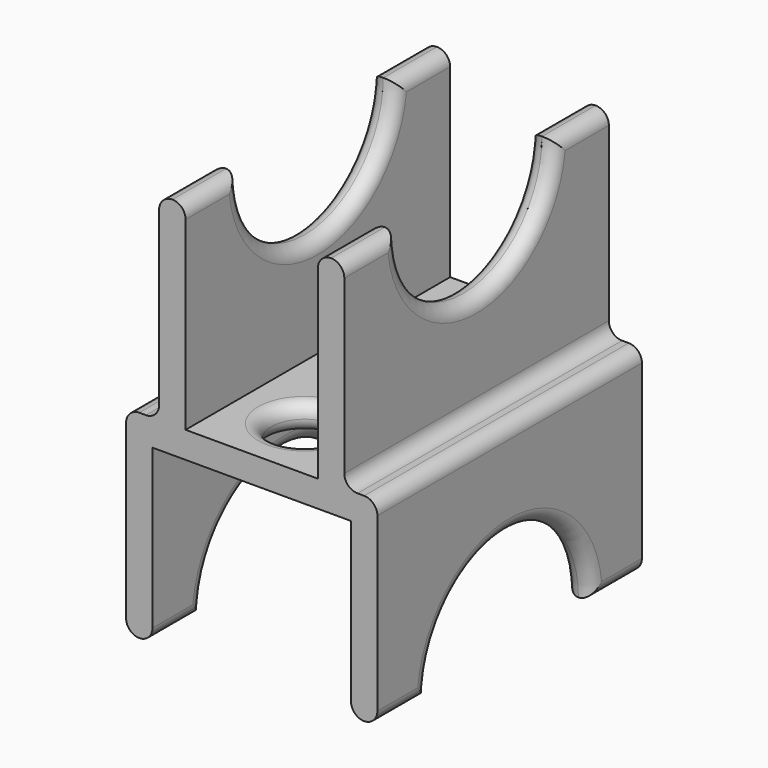
from build123d import *

# Parameters (mm, degrees)
F1_DEPTH = 63.5
F3_DEPTH = 48.261
F5_DEPTH = 41.911
F6_R     = 6.35
F7_DEPTH = 25.4
F8_R     = 2.53999


# Not quite as in the source:
# - a fillet or chamfer is up to 0.001 mm smaller than in the source, because OpenCascade refuses the exact size


with BuildPart() as f1:
    # F0 (on Front) → F1 (new body)
    with BuildSketch(Plane.XZ):
        Polygon((-10.2579592133, 51.8968305746), (-15.3379592133, 51.8968305746), (-15.3379592133, 13.7968305746), (-21.6879592133, 13.7968305746), (-21.6879592133, -24.3031694254), (-16.6079592133, -24.3031694254), (-16.6079592133, 8.7168305746), (21.4920407867, 8.7168305746), (21.4920407867, -24.3031694254), (26.5720407867, -24.3031694254), (26.5720407867, 13.7968305746), (20.2220407867, 13.7968305746), (20.2220407867, 51.8968305746), (15.1420407867, 51.8968305746), (15.1420407867, 13.7968305746), (-10.2579592133, 13.7968305746), align=None)
    extrude(amount=F1_DEPTH)

    # F2 (on face) → F3 (cut, through all)
    with BuildSketch(Plane(origin=(-21.6879592133, 0, 0), x_dir=(0, -1, 0), z_dir=(-1, 0, 0))):
        with BuildLine():
            Line((12.071813307, -24.3031694254), (51.428186693, -24.3031694254))
            ThreePointArc((51.428186693, -24.3031694254), (31.75, -4.6249827324), (12.071813307, -24.3031694254))
        make_face()
    extrude(amount=-F3_DEPTH, mode=Mode.SUBTRACT)

    # F4 (on face) → F5 (cut, through all)
    with BuildSketch(Plane(origin=(-15.3379592133, 0, 0), x_dir=(0, -1, 0), z_dir=(-1, 0, 0))):
        with BuildLine():
            ThreePointArc((12.8776709251, 51.8968305746), (31.75, 33.0245014997), (50.6223290749, 51.8968305746))
            Line((50.6223290749, 51.8968305746), (12.8776709251, 51.8968305746))
        make_face()
    extrude(amount=-F5_DEPTH, mode=Mode.SUBTRACT)

    # F6 (on face) → F7 (cut)
    with BuildSketch(Plane.XY.offset(13.7968305746)):
        with Locations((2.4420407867, -50.8)):
            Circle(F6_R)
        with Locations((2.4420407867, -12.7)):
            Circle(F6_R)
        with Locations((2.4420407867, -31.75)):
            Circle(F6_R)
    extrude(amount=-F7_DEPTH, mode=Mode.SUBTRACT)

    # F8 (radius 2.54 in the source; OpenCascade refuses exactly that, so slightly less here)
    f8_edges = [f1.edges().sort_by_distance(p)[0] for p in [
        (20.222041, -31.75, 13.796831),
        (26.572041, -31.75, 13.796831),
        (-21.687959, -31.75, 13.796831),
        (-15.337959, -31.75, 13.796831),
        (15.142041, -57.061165, 51.896831),
        (15.142041, -6.438835, 51.896831),
        (-10.257959, -6.438835, 51.896831),
        (-10.257959, -57.061165, 51.896831),
        (-15.337959, -6.438835, 51.896831),
        (-15.337959, -57.061165, 51.896831),
        (20.222041, -57.061165, 51.896831),
        (20.222041, -6.438835, 51.896831),
        (26.572041, -57.464093, -24.303169),
        (21.492041, -57.464093, -24.303169),
        (21.492041, -6.035907, -24.303169),
        (26.572041, -6.035907, -24.303169),
        (-16.607959, -6.035907, -24.303169),
        (-21.687959, -6.035907, -24.303169),
        (-21.687959, -57.464093, -24.303169),
        (-16.607959, -57.464093, -24.303169),
        (-10.257959, -31.75, 33.024501),
        (-15.337959, -31.75, 33.024501),
        (20.222041, -31.75, 33.024501),
        (15.142041, -31.75, 33.024501),
        (26.572041, -31.75, -4.624983),
        (21.492041, -31.75, -4.624983),
        (-16.607959, -31.75, -4.624983),
        (-21.687959, -31.75, -4.624983),
        (-3.907959, -50.8, 13.796831),
        (-3.907959, -31.75, 13.796831),
        (-3.907959, -12.7, 13.796831),
        (-3.907959, -50.8, 8.716831),
        (-3.907959, -31.75, 8.716831),
        (-3.907959, -12.7, 8.716831),
    ]]
    fillet(f8_edges, radius=F8_R)


solid = f1.part
